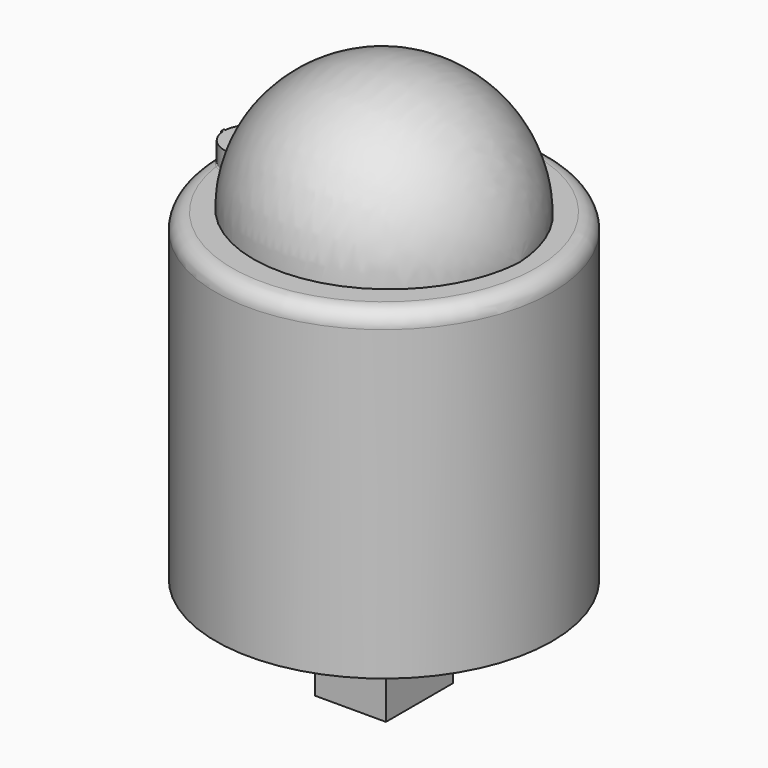
from build123d import *
from build123d import SkipClean  # not in build123d's __all__

# Parameters (mm, degrees)
F0_R      = 33.02
F1_DEPTH  = 63.5
F6_R      = 3.175
F8_W      = 13.97
F8_H      = 16.51
F9_DEPTH  = 19.05
F10_R     = 22.86
F10_R_2   = 21.844
F11_DEPTH = 1.27
F7_R      = 5.08
F12_DEPTH = 3.81
F13_R     = 0.254
F15_W     = 0.762
F15_H     = 4.3067012395
F16_DEPTH = 25.4


with BuildPart() as f1:
    # F0 (on Top) → F1 (new body)
    with BuildSketch(Plane.XY):
        Circle(F0_R)
    extrude(amount=F1_DEPTH)

    # F3 (on Front) → F4 (revolve)
    with BuildSketch(Plane.XZ):
        with BuildLine():
            Line((-26.67, 63.5), (26.67, 63.5))
            ThreePointArc((26.67, 63.5), (0, 88.9), (-26.67, 63.5))
        make_face()
    with SkipClean():  # cleaning this boolean's faces spoils the solid; the shape is the same uncleaned
        revolve(axis=Axis((0, 0, 63.5), (1, 0, 0)))

    # F6
    f6_edges = [f1.edges().sort_by_distance(p)[0] for p in [
        (-33.02, 0, 63.5),
    ]]
    fillet(f6_edges, radius=F6_R)

    # F8 (on face) → F9 (join)
    with BuildSketch(Plane(origin=(0, 0, 0), x_dir=(1, 0, 0), z_dir=(0, 0, -1))):
        Rectangle(F8_W, F8_H)
    with SkipClean():  # cleaning this boolean's faces spoils the solid; the shape is the same uncleaned
        extrude(amount=F9_DEPTH)

    # F10 (on face) → F11 (join)
    with BuildSketch(Plane(origin=(0, 0, 0), x_dir=(1, 0, 0), z_dir=(0, 0, -1))):
        Circle(F10_R)
        Circle(F10_R_2, mode=Mode.SUBTRACT)
    with SkipClean():  # cleaning this boolean's faces spoils the solid; the shape is the same uncleaned
        extrude(amount=F11_DEPTH)

    # F7 (on offset) → F12 (join, symmetric)
    with BuildSketch(Plane.XY.offset(63.5)):
        with Locations((-26.3525, 0)):
            Circle(F7_R)
    extrude(amount=F12_DEPTH, both=True)

    # F13
    f13_edges = [f1.edges().sort_by_distance(p)[0] for p in [
        (-31.4325, 0, 63.074631),
    ]]
    fillet(f13_edges, radius=F13_R)

    # F15 (on offset) → F16 (join)
    with BuildSketch(Plane.YZ.offset(-31.75)):
        with Locations((-6.0768e-06, 65.1566493803)):
            Rectangle(F15_W, F15_H)
    extrude(amount=F16_DEPTH)


solid = f1.part
